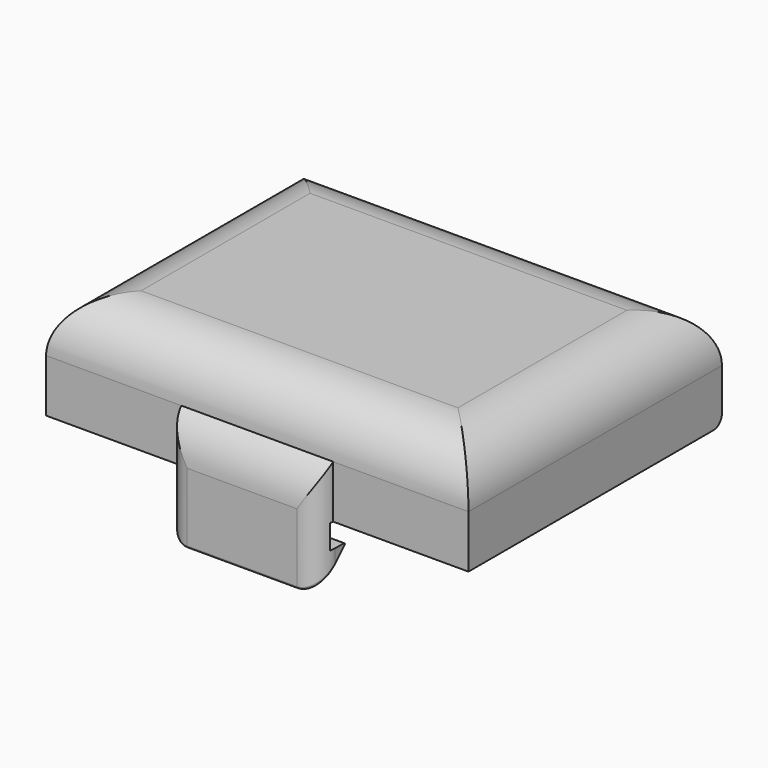
from build123d import *

# Parameters (mm, degrees)
F0_W          = 40
F0_H          = 30
F1_DEPTH      = 10
F2_R          = 5
F3_T          = -2.5
F4_W          = 27.6
F4_H          = 2.5
F5_DEPTH      = 3
F6_W          = 46.0305325687
F6_H          = 69.5610698313
F7_DEPTH      = 12.5
F8_R          = 0.55
F9_DEPTH      = 0.55
F10_R         = 0.54999
F11_R         = 1
F13_W         = 14.4
F13_H         = 12
F14_DEPTH     = 1.8
F16_DEPTH     = 25
F17_T4_DEPTH  = 20.8
F17_T9_DEPTH  = 20.8
F17_T14_DEPTH = 20.8
F17_T19_DEPTH = 20.8
F18_T1_DEPTH  = 29.6093727123
F19_R         = 0.2


# Not quite as in the source:
# - a fillet or chamfer that OpenCascade refuses, or shapes differently, is made with other operations: its cross-section is extruded or revolved along the edge and cut away or added
# - a fillet or chamfer is up to 0.001 mm smaller than in the source, because OpenCascade refuses the exact size


with BuildPart() as f1:
    # F0 (on Top) → F1 (new body)
    with BuildSketch(Plane.XY):
        Rectangle(F0_W, F0_H)
    extrude(amount=F1_DEPTH)

    # F2
    f2_edges = [f1.edges().sort_by_distance(p)[0] for p in [
        (20, 0, 10),
        (0, 15, 10),
        (-20, 0, 10),
        (0, -15, 10),
    ]]
    fillet(f2_edges, radius=F2_R)

    # F3
    f3_openings = [f1.faces().sort_by_distance(p)[0] for p in [
        (0, 0, 0),
    ]]
    offset(amount=F3_T, openings=f3_openings)

    # F4 (on Top) → F5 (join)
    with BuildSketch(Plane.XY):
        with Locations((0, 13.75)):
            Rectangle(F4_W, F4_H)
    extrude(amount=-F5_DEPTH)

    # F6 (on Top) → F7 (cut, symmetric)
    with BuildSketch(Plane.XY):
        with Locations((23.0152662843, -8.845419623)):
            Rectangle(F6_W, F6_H)
    extrude(amount=F7_DEPTH, both=True, mode=Mode.SUBTRACT)

    # F8 (on face) → F9 (join)
    with BuildSketch(Plane(origin=(-13.8, 0, 0), x_dir=(0, -1, 0), z_dir=(-1, 0, 0))):
        with Locations((-13.75, -1.5)):
            Circle(F8_R)
    extrude(amount=F9_DEPTH)

    # F10 (radius 0.55 in the source; OpenCascade refuses exactly that, so slightly less here)
    f10_edges = [f1.edges().sort_by_distance(p)[0] for p in [
        (-14.35, 14.3, -1.5),
    ]]
    fillet(f10_edges, radius=F10_R)

    # F11
    f11_edges = [f1.edges().sort_by_distance(p)[0] for p in [
        (-6.9, 15, -3),
        (-6.9, 12.5, -3),
        (-16.9, 15, 0),
        (-15.65, 12.5, 0),
    ]]
    fillet(f11_edges, radius=F11_R)

    # F12: F1 across plane


with BuildPart() as f1_1:
    add(f1.part)
    add(f1.part.mirror(Plane.YZ))

    # F13 (on face) → F14 (join, symmetric)
    with BuildSketch(Plane.XZ.offset(15)):
        with Locations((0, -1)):
            Rectangle(F13_W, F13_H)
    extrude(amount=F14_DEPTH, both=True)

    # F15 (on face) → F16 (cut)
    with BuildSketch(Plane(origin=(-7.2, 0, 0), x_dir=(0, -1, 0), z_dir=(-1, 0, 0))):
        Polygon((15.3, 0), (15, 0), (13.2, 0), (13.2, -7), (16.8, -7), (16.8, -5.8), (13.3, -2.3), (15.3, -2.3), align=None)
    extrude(amount=-F16_DEPTH, mode=Mode.SUBTRACT)

    # F17: fillet of radius 2 on 2 edges, made by hand


with BuildPart() as f17_tool2:
    # F17_s3 → F17_t4 (new body)
    with BuildSketch(Plane.XY.offset(10)):
        with BuildLine():
            ThreePointArc((-5.2, -16.8), (-6.6142135624, -16.2142135624), (-7.2, -14.8))
            Line((-7.2, -14.8), (-7.2, -16.8))
            Line((-7.2, -16.8), (-5.2, -16.8))
        make_face()
    extrude(amount=-F17_T4_DEPTH)

    split(bisect_by=Plane.XZ.offset(15), keep=Keep.TOP)


with BuildPart() as f1_2:
    add(f1_1.part)

    # F17_t1: cut F17_tool2
    add(f17_tool2.part, mode=Mode.SUBTRACT)


with BuildPart() as f17_tool7:
    # F17_s8 → F17_t9 (new body)
    with BuildSketch(Plane.XY.offset(10)):
        with BuildLine():
            ThreePointArc((-5.2, -16.8), (-6.6142135624, -16.2142135624), (-7.2, -14.8))
            Line((-7.2, -14.8), (-7.2, -16.8))
            Line((-7.2, -16.8), (-5.2, -16.8))
        make_face()
    extrude(amount=-F17_T9_DEPTH)

    split(bisect_by=Plane.XY, keep=Keep.BOTTOM)


with BuildPart() as f1_3:
    add(f1_2.part)

    # F17_t6: cut F17_tool7
    add(f17_tool7.part, mode=Mode.SUBTRACT)


with BuildPart() as f17_tool12:
    # F17_s13 → F17_t14 (new body)
    with BuildSketch(Plane.XY.offset(-10.8)):
        with BuildLine():
            ThreePointArc((5.2, -16.8), (6.6142135624, -16.2142135624), (7.2, -14.8))
            Line((7.2, -14.8), (7.2, -16.8))
            Line((7.2, -16.8), (5.2, -16.8))
        make_face()
    extrude(amount=F17_T14_DEPTH)

    split(bisect_by=Plane.XZ.offset(15), keep=Keep.TOP)


with BuildPart() as f1_4:
    add(f1_3.part)

    # F17_t11: cut F17_tool12
    add(f17_tool12.part, mode=Mode.SUBTRACT)


with BuildPart() as f17_tool17:
    # F17_s18 → F17_t19 (new body)
    with BuildSketch(Plane.XY.offset(-10.8)):
        with BuildLine():
            ThreePointArc((5.2, -16.8), (6.6142135624, -16.2142135624), (7.2, -14.8))
            Line((7.2, -14.8), (7.2, -16.8))
            Line((7.2, -16.8), (5.2, -16.8))
        make_face()
    extrude(amount=F17_T19_DEPTH)

    split(bisect_by=Plane.XY, keep=Keep.BOTTOM)


with BuildPart() as f1_5:
    add(f1_4.part)

    # F17_t16: cut F17_tool17
    add(f17_tool17.part, mode=Mode.SUBTRACT)

    # F18: fillet of radius 5 on 1 edges, made by hand

    # F18_s2 → F18_t1 (cut)
    with BuildSketch(Plane.YZ.offset(-14.8046863561)):
        with BuildLine():
            ThreePointArc((-16.8, 1.1581254575), (-16.3276925691, 3.2794458011), (-15, 5))
            Line((-15, 5), (-16.8, 5))
            Line((-16.8, 5), (-16.8, 1.1581254575))
        make_face()
    extrude(amount=F18_T1_DEPTH, mode=Mode.SUBTRACT)

    # F19
    f19_edges = [f1_5.edges().sort_by_distance(p)[0] for p in [
        (-7.2, -14.05, -3.05),
        (0, -13.3, -2.3),
        (7.2, -14.05, -3.05),
        (7.197495, -14.900063, -3.900063),
        (6.65083, -16.176624, -5.176624),
        (0, -16.8, -5.8),
        (-6.65083, -16.176624, -5.176624),
        (-7.197495, -14.900063, -3.900063),
    ]]
    fillet(f19_edges, radius=F19_R)


solid = f1_5.part
